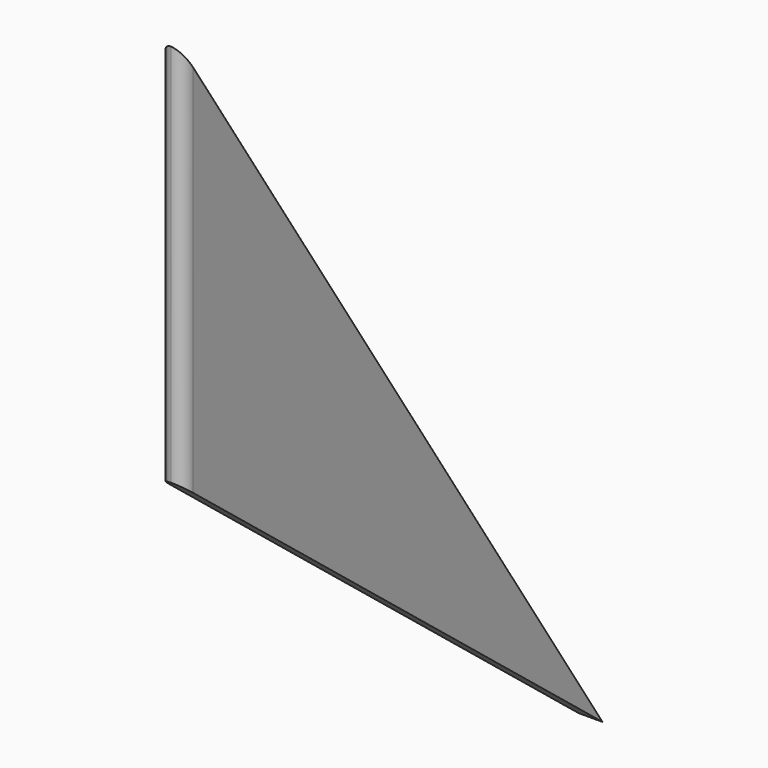
from build123d import *

# Parameters (mm, degrees)
F1_DEPTH    = 2.5
F2_T1_DEPTH = 46.75


# Not quite as in the source:
# - a fillet or chamfer that OpenCascade refuses, or shapes differently, is made with other operations: its cross-section is extruded or revolved along the edge and cut away or added


with BuildPart() as f1:
    # F0 (on Right) → F1 (new body)
    with BuildSketch(Plane.YZ):
        Polygon((0, 40), (0, 0), (54.643732486, -43.75), align=None)
    extrude(amount=F1_DEPTH)

    # F2: fillet of radius 1.35 on 2 edges, made by hand

    # F2_s2 → F2_t1 (cut)
    with BuildSketch(Plane.XY.offset(-3.375)):
        with BuildLine():
            ThreePointArc((1.15, 0), (2.1045941546, 0.3954058454), (2.5, 1.35))
            Line((2.5, 1.35), (2.5, 0))
            Line((2.5, 0), (1.15, 0))
        make_face()
        with BuildLine():
            ThreePointArc((1.35, 0), (0.3954058454, 0.3954058454), (0, 1.35))
            Line((0, 1.35), (0, 0))
            Line((0, 0), (1.35, 0))
        make_face()
    extrude(amount=F2_T1_DEPTH, mode=Mode.SUBTRACT)


solid = f1.part
